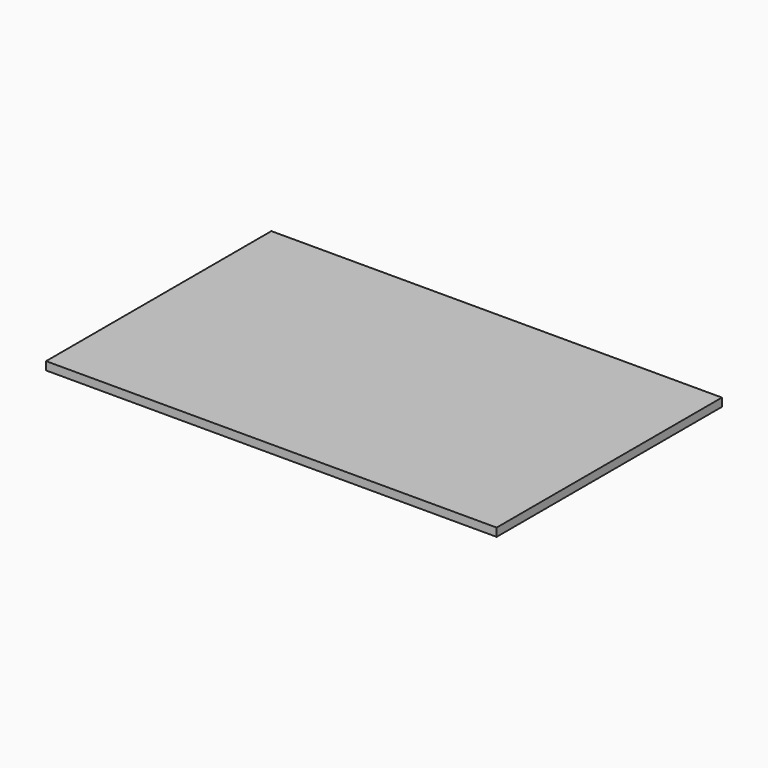
from build123d import *

# Parameters (mm, degrees)
F0_W     = 1219.2
F0_H     = 762
F1_DEPTH = 22.225


# Not quite as in the source:
# - a length typed as a fraction of an inch, garbled in the dataset ("3 / 203.2 mm" for 3/8 in), is restored


with BuildPart() as f1:
    # F0 (on Top) → F1 (new body)
    with BuildSketch(Plane.XY):
        with Locations((-70.9174834192, 195.97042596)):
            Rectangle(F0_W, F0_H)
    extrude(amount=F1_DEPTH)


solid = f1.part
